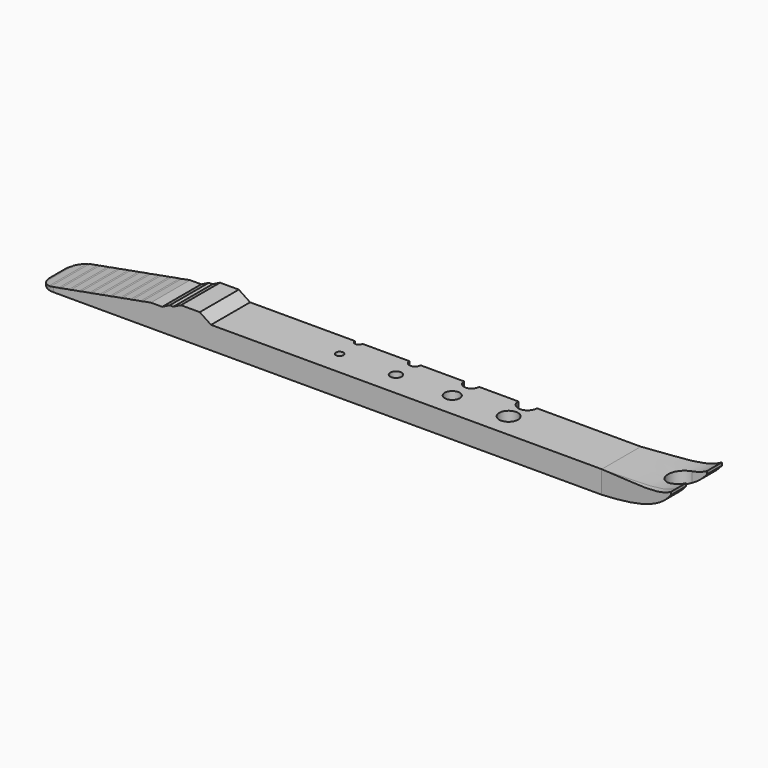
from build123d import *

# Parameters (mm, degrees)
F0_R          = 1
F0_R_2        = 1.5
F0_R_3        = 2
F1_DEPTH      = 6
F3_DEPTH      = 8
F5_DEPTH      = 25
F5_DEPTH_BACK = 25
F7_DEPTH      = 25
F9_DEPTH      = 13


# Not quite as in the source:
# - a feature names something its author has since deleted; it is built from what else it names


with BuildPart() as f1:
    # F0 (on Top) → F1 (new body)
    with BuildSketch(Plane.XY):
        with BuildLine():
            Line((-42.1966487169, -12.8954221606), (-42.1966487169, -25.8954221606))
            Line((-42.1966487169, -25.8954221606), (17.9292613268, -25.8954221606))
            Line((17.9292613268, -25.8954221606), (47.9292613268, -25.8954221606))
            Line((47.9292613268, -25.8954221606), (47.9292613268, -12.8954221606))
            Line((47.9292613268, -12.8954221606), (20.3033512831, -12.8954221606))
            ThreePointArc((20.3033512831, -12.8954221606), (17.8033512831, -15.3954221606), (15.3033512831, -12.8954221606))
            Line((15.3033512831, -12.8954221606), (4.8663063049, -12.8954221606))
            ThreePointArc((4.8663063049, -12.8954221606), (2.8663063049, -14.8954221606), (0.8663063049, -12.8954221606))
            Line((0.8663063049, -12.8954221606), (-10.6966487169, -12.8954221606))
            ThreePointArc((-10.6966487169, -12.8954221606), (-12.1966487169, -14.3954221606), (-13.6966487169, -12.8954221606))
            Line((-13.6966487169, -12.8954221606), (-26.1966487169, -12.8954221606))
            ThreePointArc((-26.1966487169, -12.8954221606), (-27.1966487169, -13.8954221606), (-28.1966487169, -12.8954221606))
            Line((-28.1966487169, -12.8954221606), (-42.1966487169, -12.8954221606))
        make_face()
        with Locations((-27.0707386732, -19.3954221606)):
            Circle(F0_R, mode=Mode.SUBTRACT)
        with Locations((-12.0707386732, -19.3954221606)):
            Circle(F0_R_2, mode=Mode.SUBTRACT)
        with Locations((2.9292613268, -19.3954221606)):
            Circle(F0_R_3, mode=Mode.SUBTRACT)
        with BuildLine():
            ThreePointArc((20.4292613268, -19.3954221606), (19.6970282798, -21.1631891136), (17.9292613268, -21.8954221606))
            ThreePointArc((17.9292613268, -21.8954221606), (16.1614943738, -17.6276552077), (20.4292613268, -19.3954221606))
        make_face(mode=Mode.SUBTRACT)
        with BuildLine():
            ThreePointArc((-102.1092408178, -21.9157785711), (-100.9305134828, -24.7310372299), (-98.109292616, -25.8954221606))
            Line((-98.109292616, -25.8954221606), (-42.1966487169, -25.8954221606))
            Line((-42.1966487169, -25.8954221606), (-42.1966487169, -12.8954221606))
            Line((-42.1966487169, -12.8954221606), (-98.1347384587, -12.8954221606))
            ThreePointArc((-98.1347384587, -12.8954221606), (-100.9703535279, -14.0742012939), (-102.1346866604, -16.9157785711))
            Line((-102.1346866604, -16.9157785711), (-102.1092408178, -21.9157785711))
        make_face()
    extrude(amount=F1_DEPTH)

    # F2 (on face) → F3 (join)
    with BuildSketch(Plane(origin=(0, 0, 0), x_dir=(1, 0, 0), z_dir=(0, 0, -1))):
        with BuildLine():
            Line((47.9292613268, 25.8954221606), (47.9292613268, 12.8954221606))
            Line((47.9292613268, 12.8954221606), (67.9292613268, 10.8954221606))
            Line((67.9292613268, 10.8954221606), (67.9292613268, 15.8954221606))
            Line((67.9292613268, 15.8954221606), (63.9292613268, 15.8954221606))
            ThreePointArc((63.9292613268, 15.8954221606), (60.4292613268, 19.3954221606), (63.9292613268, 22.8954221606))
            Line((63.9292613268, 22.8954221606), (67.9292613268, 22.8954221606))
            Line((67.9292613268, 22.8954221606), (67.9292613268, 27.8954221606))
            Line((67.9292613268, 27.8954221606), (47.9292613268, 25.8954221606))
        make_face()
    extrude(amount=-F3_DEPTH)

    # F4 (on face) → F5 (cut, two sides)
    with BuildSketch(Plane.XZ.offset(25.8954221606)) as f5_sk:
        with BuildLine():
            Line((46.540889889, 6), (47.9292613268, 6))
            add(Edge.make_bspline(
                [(47.9292613268, 6), (56.2153583024, 6.3852668293), (63.4993069571, 5.4990063105), (67.9292613268, 8)],
                knots=[0, 0, 0, 0, 0.5891408943, 0.5891408943, 0.5891408943, 0.5891408943], degree=3))
            add(Edge.make_bspline(
                [(67.9292613268, 8), (68.2487173743, 8.1803534511), (68.5533319552, 8.3783214507), (68.8425013824, 8.5922158425)],
                knots=[0.5891408943, 0.5891408943, 0.5891408943, 0.5891408943, 0.6316254451, 0.6316254451, 0.6316254451, 0.6316254451], degree=3))
            add(Edge.make_bspline(
                [(68.8425013824, 8.5922158425), (70.5907749543, 11.5561393325), (71.3452296215, 15.074575864), (72.5077323308, 15.8934572506)],
                knots=[0.4687959677, 0.4687959677, 0.4687959677, 0.4687959677, 0.7089887452, 0.7089887452, 0.7089887452, 0.7089887452], degree=3))
            add(Edge.make_bspline(
                [(72.5077323308, 15.8934572506), (72.5145030374, 15.8982266206), (72.5212875857, 15.9029044167), (72.5280862528, 15.9074899958)],
                knots=[0.7089887452, 0.7089887452, 0.7089887452, 0.7089887452, 0.710387688, 0.710387688, 0.710387688, 0.710387688], degree=3))
            Line((72.5280862528, 15.9074899958), (72.5280862528, 21.5322930813))
            Line((72.5280862528, 21.5322930813), (47.9292613268, 21.5322930813))
            Line((47.9292613268, 21.5322930813), (46.540889889, 21.5322930813))
            Line((46.540889889, 21.5322930813), (46.540889889, 6))
        make_face()
        with BuildLine():
            add(Edge.make_bspline(
                [(47.9292613268, 0), (56.4914134681, 0.9755749136), (64.1655487647, 2.3840198172), (67.9292613268, 7.2357458994)],
                knots=[0, 0, 0, 0, 0.4306699839, 0.4306699839, 0.4306699839, 0.4306699839], degree=3))
            Line((47.9292613268, 0), (47.9292613268, -3.928697668))
            Line((47.9292613268, -3.928697668), (72.5280862528, -3.928697668))
            Line((72.5280862528, -3.928697668), (72.5280862528, 15.9074899958))
            add(Edge.make_bspline(
                [(72.5077323308, 15.8934572506), (72.5145030374, 15.8982266206), (72.5212875857, 15.9029044167), (72.5280862528, 15.9074899958)],
                knots=[0.7089887452, 0.7089887452, 0.7089887452, 0.7089887452, 0.710387688, 0.710387688, 0.710387688, 0.710387688], degree=3))
            add(Edge.make_bspline(
                [(68.8425013824, 8.5922158425), (71.1489726079, 10.2982788409), (72.4728284355, 13.0175734735), (72.5077323308, 15.8934572506)],
                knots=[0.6316254451, 0.6316254451, 0.6316254451, 0.6316254451, 0.9704904314, 0.9704904314, 0.9704904314, 0.9704904314], degree=3))
            add(Edge.make_bspline(
                [(67.9292613268, 7.2357458994), (68.2624520517, 7.6652553541), (68.5649965775, 8.1217499937), (68.8425013824, 8.5922158425)],
                knots=[0.4306699839, 0.4306699839, 0.4306699839, 0.4306699839, 0.4687959677, 0.4687959677, 0.4687959677, 0.4687959677], degree=3))
        make_face()
    extrude(amount=-F5_DEPTH, mode=Mode.SUBTRACT)
    extrude(f5_sk.sketch, amount=F5_DEPTH_BACK, mode=Mode.SUBTRACT)

    # F6 (on face) → F7 (cut)
    with BuildSketch(Plane.XZ.offset(25.8954221606)):
        Polygon((-110.3505343199, 7.7635785565), (-102.109292616, 0), (-102.109292616, 0.5), (-101.609292616, 0.5), (-101.609292616, 0.5916666667), (-99.3820198888, 1), (-98.8820198888, 1), (-98.8820198888, 1.0916666667), (-96.6547471615, 1.5), (-96.1547471615, 1.5), (-96.1547471615, 1.5916666667), (-93.9274744342, 2), (-93.4274744342, 2), (-93.4274744342, 2.0916666667), (-91.200201707, 2.5), (-90.700201707, 2.5), (-90.700201707, 2.5916666667), (-88.4729289797, 3), (-87.9729289797, 3), (-87.9729289797, 3.0916666667), (-85.7456562524, 3.5), (-85.2456562524, 3.5), (-85.2456562524, 3.5916666667), (-83.0183835251, 4), (-82.5183835251, 4), (-82.5183835251, 4.0916666667), (-80.2911107979, 4.5), (-79.7911107979, 4.5), (-79.7911107979, 4.5916666667), (-77.5638380706, 5), (-77.0638380706, 5), (-77.0638380706, 5.0916666667), (-74.8365653433, 5.5), (-74.3365653433, 5.5), (-74.3365653433, 5.5916666667), (-72.109292616, 6), (-71.3678747416, 6.6357897595), (-76.816663146, 6.5958285704), (-98.5576808453, 7.7635785565), align=None)
    extrude(amount=-F7_DEPTH, mode=Mode.SUBTRACT)

    # F8 (on face) → F9 (join)
    with BuildSketch(Plane.XZ.offset(25.8954221606)):
        Polygon((-67.109292616, 7), (-69.109292616, 6), (-67.109292616, 6), (-56.109292616, 6), (-59.109292616, 8), (-64.109292616, 8), (-66.109292616, 7), align=None)
    extrude(amount=-F9_DEPTH)


solid = f1.part
